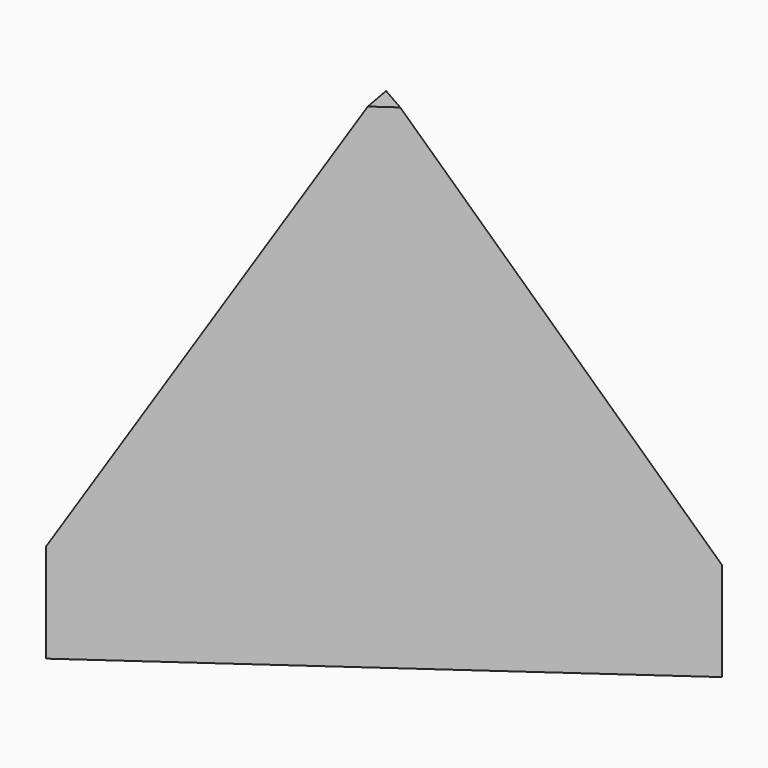
from build123d import *

# Parameters (mm, degrees)
F1_DEPTH    = 2
F2_DEPTH    = 15
F3_T1_DEPTH = 65.3920789545
F3_T3_DEPTH = 65.4809656857


# Not quite as in the source:
# - a fillet or chamfer that OpenCascade refuses, or shapes differently, is made with other operations: its cross-section is extruded or revolved along the edge and cut away or added


with BuildPart() as f1:
    # F0 (on Top) → F1 (new body)
    with BuildSketch(Plane.XY):
        Polygon((6.2144221197, 1.7468538459), (-7.3403550955, 9.487123932), (-4.5410526356, -5.9592496019), align=None)
        Polygon((9.1590517926, 0.0653633566), (6.2144221197, 1.7468538459), (-4.5410526356, -5.9592496019), (-3.9522281139, -9.2083459887), align=None)
    extrude(amount=F1_DEPTH)

    # F0 (on Top) → F2 (join)
    with BuildSketch(Plane.XY):
        Polygon((9.1590517926, 0.0653633566), (6.2144221197, 1.7468538459), (-4.5410526356, -5.9592496019), (-3.9522281139, -9.2083459887), align=None)
    extrude(amount=F2_DEPTH)

    # F3: chamfer of 12 x 6.9282032303 on 2 edges, made by hand

    # F3_s2 → F3_t1 (cut)
    with BuildSketch(Plane(origin=(-4.6347910576, 25.5744832693, 0), x_dir=(0, 0, 1), z_dir=(0.1783224727, -0.9839721011, 0))):
        Polygon((3, 5.5309372275), (15, -1.3972660027), (15, 5.5309372275), align=None)
    extrude(amount=F3_T1_DEPTH, mode=Mode.SUBTRACT)

    # F3_s4 → F3_t3 (cut)
    with BuildSketch(Plane(origin=(33.8378902633, -19.3226642995, 0), x_dir=(0, 0, 1), z_dir=(-0.8683898362, 0.4958821356, 0))):
        Polygon((15, -2.3296321932), (3, 4.5985710371), (15, 4.5985710371), align=None)
    extrude(amount=F3_T3_DEPTH, mode=Mode.SUBTRACT)


solid = f1.part
